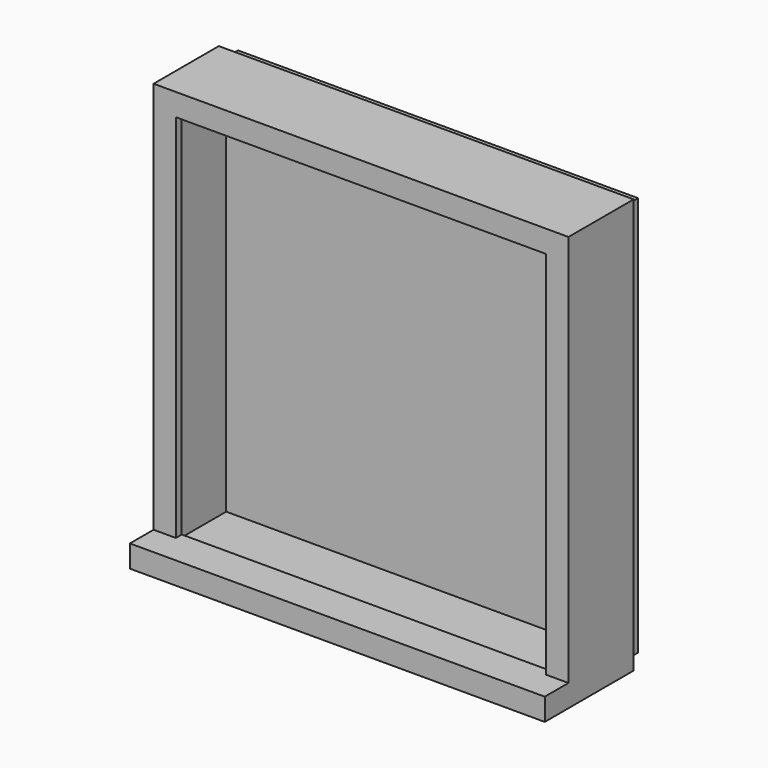
from build123d import *

# Parameters (mm, degrees)
F0_W      = 56
F0_H      = 56
F0_W_2    = 54
F0_H_2    = 54
F1_DEPTH  = 10
F2_W      = 56
F2_H      = 56
F2_W_2    = 54
F2_H_2    = 54
F2_W_3    = 50
F2_H_3    = 50
F3_DEPTH  = 1
F4_DEPTH  = 2
F5_W      = 5
F5_H      = 5
F6_DEPTH  = 5
F8_DEPTH  = 4
F10_DEPTH = 2


# Not quite as in the source:
# - a feature of the source that left no trace in its solid (it failed there, or was rolled back) is left out


with BuildPart() as f1:
    # F0 (on Front) → F1 (new body)
    with BuildSketch(Plane.XZ):
        Rectangle(F0_W, F0_H)
        Rectangle(F0_W_2, F0_H_2, mode=Mode.SUBTRACT)
    extrude(amount=F1_DEPTH)

    # F2 (on face) → F3 (join)
    with BuildSketch(Plane.XZ.offset(10)):
        Rectangle(F2_W, F2_H)
        Rectangle(F2_W_2, F2_H_2, mode=Mode.SUBTRACT)
        Rectangle(F2_W_2, F2_H_2)
        Rectangle(F2_W_3, F2_H_3, mode=Mode.SUBTRACT)
    extrude(amount=F3_DEPTH)

    # F7 (on face) → F8 (join)
    with BuildSketch(Plane.XZ.offset(11)):
        Polygon((-28, -25), (-28, -28), (28, -28), (28, -25), (25, -25), (-25, -25), align=None)
    extrude(amount=F8_DEPTH)

    # F9 (on face) → F10 (cut)
    with BuildSketch(Plane(origin=(0, 0, -28), x_dir=(1, 0, 0), z_dir=(0, 0, -1))):
        Polygon((-26.9533358514, 10), (-23.9533358514, 10), (-23.9533358514, 14.5), (-28, 14.5), (-28, 11.5), (-26.9533358514, 11.5), align=None)
    extrude(amount=-F10_DEPTH, mode=Mode.SUBTRACT)


with BuildPart() as f4:
    # F0 (on Front) → F4 (new body)
    with BuildSketch(Plane.XZ):
        Rectangle(F0_W_2, F0_H_2)
    extrude(amount=-F4_DEPTH)

    # F5 (on face) → F6 (join)
    with BuildSketch(Plane(origin=(0, 2, 0), x_dir=(-1, 0, 0), z_dir=(0, 1, 0))):
        Rectangle(F5_W, F5_H)
    extrude(amount=F6_DEPTH)


solid = Compound([f1.part, f4.part])
